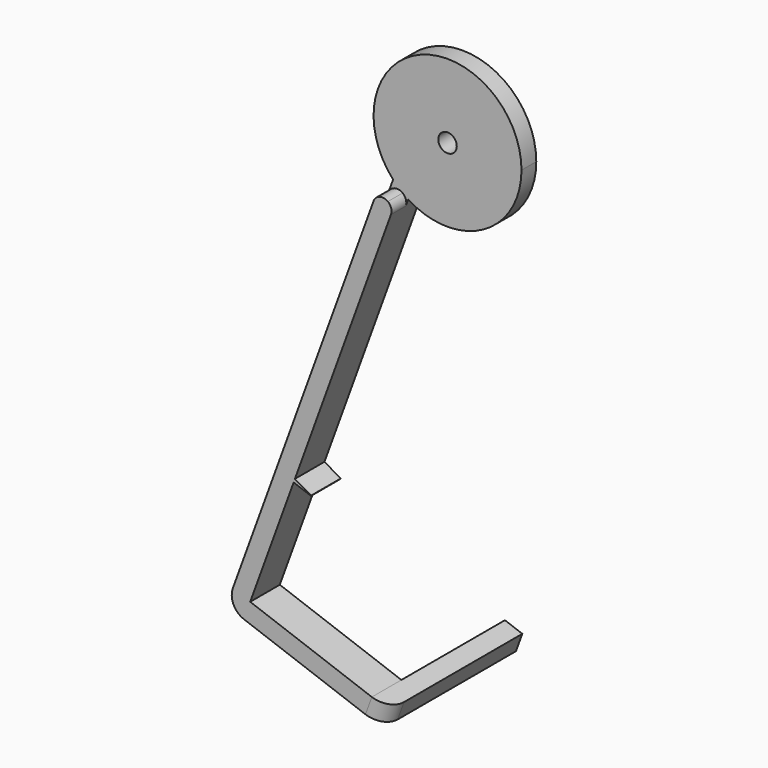
from build123d import *

# Parameters (mm, degrees)
F0_R        = 2.5
F1_DEPTH    = 5
F2_DEPTH    = 10
F3_R        = 2.49999
F4_T1_DEPTH = 35
F4_T3_DEPTH = 30
F5_SIZE2    = 0.881625
F5_SIZE     = 4.99999
F6_DEPTH    = 35


# Not quite as in the source:
# - a fillet or chamfer that OpenCascade refuses, or shapes differently, is made with other operations: its cross-section is extruded or revolved along the edge and cut away or added
# - a fillet or chamfer is up to 0.001 mm smaller than in the source, because OpenCascade refuses the exact size


with BuildPart() as f1:
    # F0 (on Front) → F1 (new body)
    with BuildSketch(Plane.XZ):
        with BuildLine():
            ThreePointArc((20, 33.8170940264), (-7.2600924867, 52.4528407806), (-14.7291057085, 20.287369527))
            ThreePointArc((-14.7291057085, 20.287369527), (-12.8011117725, 18.4505219497), (-10.6461806987, 16.8860917959))
            ThreePointArc((-10.6461806987, 16.8860917959), (9.671514515, 16.3110434442), (20, 33.8170940264))
        make_face()
        with Locations((0, 33.8170940264)):
            Circle(F0_R, mode=Mode.SUBTRACT)
        with BuildLine():
            Line((-42.3206788698, -55.5198547009), (-37.6222157658, -57.2299554175))
            Line((-37.6222157658, -57.2299554175), (-37.2801956225, -56.2902627967))
            Line((-37.2801956225, -56.2902627967), (-10.6461806987, 16.8860917959))
            ThreePointArc((-10.6461806987, 16.8860917959), (-12.8011117725, 18.4505219497), (-14.7291057085, 20.287369527))
            Line((-14.7291057085, 20.287369527), (-42.3206788698, -55.5198547009))
        make_face()
        Polygon((-37.2801956225, -56.2902627967), (-37.6222157658, -57.2299554175), (-32.9237526619, -58.9400561341), (-32.5817325186, -58.0003635134), align=None)
        Polygon((-49.362959087, -89.48738258), (-37.6222157658, -57.2299554175), (-42.3206788698, -55.5198547009), (-55.7715229075, -92.4757449673), (-51.0730598036, -94.1858456839), align=None)
        Polygon((-16.4737173595, -101.4580875964), (-49.362959087, -89.48738258), (-51.0730598036, -94.1858456839), (-18.1838180761, -106.1565507003), align=None)
        Polygon((-11.7752542555, -103.168188313), (-16.4737173595, -101.4580875964), (-18.1838180761, -106.1565507003), (-13.4853549722, -107.8666514169), align=None)
    extrude(amount=F1_DEPTH)

    # F0 (on Front) → F2 (join)
    with BuildSketch(Plane.XZ):
        with BuildLine():
            Line((-42.3206788698, -55.5198547009), (-37.6222157658, -57.2299554175))
            Line((-37.6222157658, -57.2299554175), (-37.2801956225, -56.2902627967))
            Line((-37.2801956225, -56.2902627967), (-10.6461806987, 16.8860917959))
            ThreePointArc((-10.6461806987, 16.8860917959), (-12.8011117725, 18.4505219497), (-14.7291057085, 20.287369527))
            Line((-14.7291057085, 20.287369527), (-42.3206788698, -55.5198547009))
        make_face()
        Polygon((-49.362959087, -89.48738258), (-37.6222157658, -57.2299554175), (-42.3206788698, -55.5198547009), (-55.7715229075, -92.4757449673), (-51.0730598036, -94.1858456839), align=None)
        Polygon((-16.4737173595, -101.4580875964), (-49.362959087, -89.48738258), (-51.0730598036, -94.1858456839), (-18.1838180761, -106.1565507003), align=None)
        Polygon((-11.7752542555, -103.168188313), (-16.4737173595, -101.4580875964), (-18.1838180761, -106.1565507003), (-13.4853549722, -107.8666514169), align=None)
        Polygon((-37.2801956225, -56.2902627967), (-37.6222157658, -57.2299554175), (-32.9237526619, -58.9400561341), (-32.5817325186, -58.0003635134), align=None)
    extrude(amount=F2_DEPTH)

    # F3 (radius 2.5 in the source; OpenCascade refuses exactly that, so slightly less here)
    f3_edges = [f1.edges().sort_by_distance(p)[0] for p in [
        (-10.646181, -7.5, 16.886092),
        (-14.729106, -7.5, 20.28737),
    ]]
    fillet(f3_edges, radius=F3_R)

    # F4: fillet of radius 5 on 2 edges, made by hand

    # F4_s2 → F4_t1 (cut)
    with BuildSketch(Plane.XZ.offset(-12.5)):
        with BuildLine():
            ThreePointArc((-54.0614221909, -87.7772818634), (-53.8944980222, -91.6004738887), (-51.0730598036, -94.1858456839))
            Line((-51.0730598036, -94.1858456839), (-55.7715229075, -92.4757449673))
            Line((-55.7715229075, -92.4757449673), (-54.0614221909, -87.7772818634))
        make_face()
    extrude(amount=F4_T1_DEPTH, mode=Mode.SUBTRACT)

    # F4_s4 → F4_t3 (cut)
    with BuildSketch(Plane(origin=(-40.5204121723, 0, -111.3289174704), x_dir=(0, 1, 0), z_dir=(0.3420201433, 0, 0.9396926208))):
        with BuildLine():
            ThreePointArc((-10, -19.2204790217), (-8.5355339059, -22.7560129276), (-5, -24.2204790217))
            Line((-5, -24.2204790217), (-10, -24.2204790217))
            Line((-10, -24.2204790217), (-10, -19.2204790217))
        make_face()
    extrude(amount=F4_T3_DEPTH, mode=Mode.SUBTRACT)

    # F5 (size 5 and 0.8816349035 in the source; OpenCascade refuses exactly that, so slightly less here)
    f5_edges = [f1.edges().sort_by_distance(p)[0] for p in [
        (-32.581733, -5, -58.000364),
    ]]
    chamfer(f5_edges, length=F5_SIZE, length2=F5_SIZE2)

    # F0 (on Front) → F6 (join)
    with BuildSketch(Plane.XZ):
        Polygon((-11.7752542555, -103.168188313), (-16.4737173595, -101.4580875964), (-18.1838180761, -106.1565507003), (-13.4853549722, -107.8666514169), align=None)
    extrude(amount=-F6_DEPTH)


solid = f1.part
